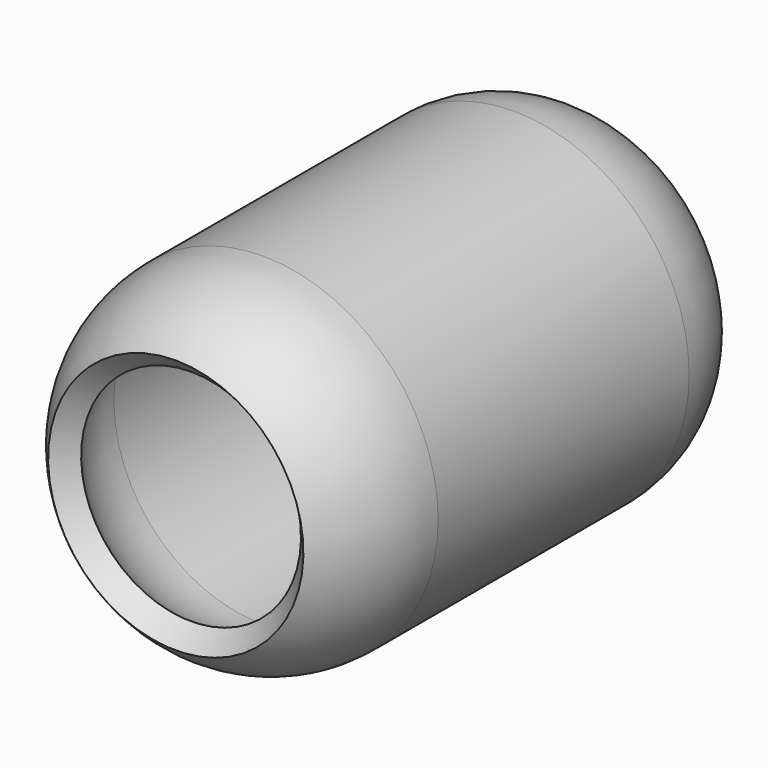
from build123d import *


# Not quite as in the source:
# - the program builds the solid bodies; features that only make, move or delete a surface that nothing else refers to are left out


with BuildPart() as f1:
    # F0 (on Right) → F1 (revolve)
    with BuildSketch(Plane.YZ):
        with BuildLine():
            ThreePointArc((-85.1584672928, 37.4418093443), (-71.2460039927, 47.3150231752), (-54.5459464192, 50.8))
            Line((-54.5459464192, 50.8), (52.3195825517, 50.8))
            ThreePointArc((52.3195825517, 50.8), (64.2327817533, 48.4117935532), (74.3049383163, 41.6162429929))
            Line((74.3049383163, 41.6162429929), (80.6286030972, 47.8647119045))
            ThreePointArc((80.6286030972, 47.8647119045), (67.6593843985, 56.6148718968), (52.3195825517, 59.69))
            Line((52.3195825517, 59.69), (-54.5459464192, 59.69))
            ThreePointArc((-54.5459464192, 59.69), (-74.8015101461, 55.4630582753), (-91.6759901132, 43.487799444))
            Line((-91.6759901132, 43.487799444), (-85.1584672928, 37.4418093443))
        make_face()
    revolve(axis=Axis((0, 0.417444855, 0), (0, 1, 0)))


solid = f1.part
